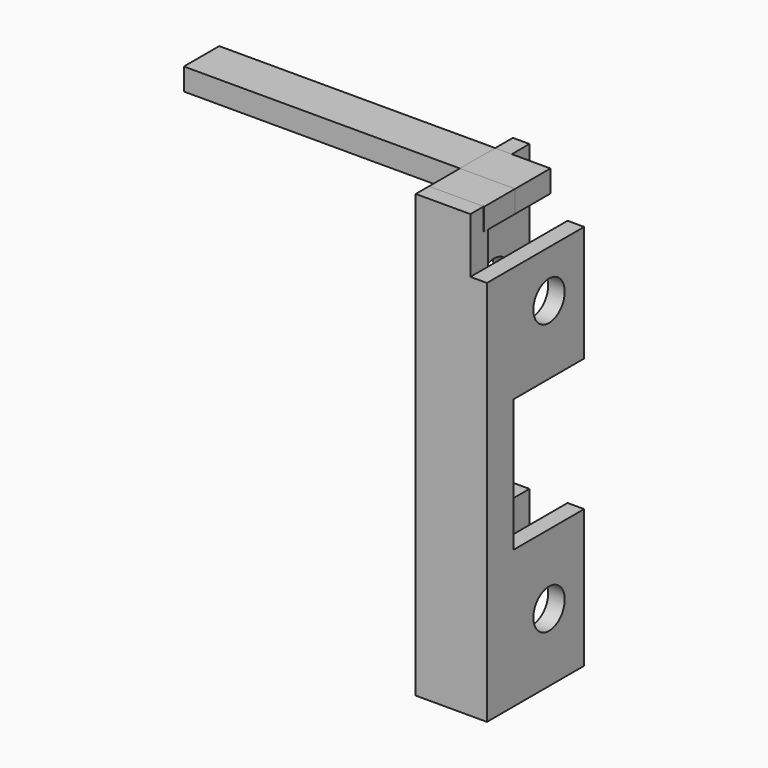
from build123d import *

# Parameters (mm, degrees)
F1_DEPTH  = 70
F2_R      = 3.55
F3_DEPTH  = 12.901
F5_DEPTH  = 10
F6_W      = 8
F6_H      = 4
F7_DEPTH  = 50
F8_W      = 9.9
F8_H      = 24
F8_W_2    = 3
F9_DEPTH  = 16
F10_DEPTH = 10
F11_DEPTH = 7


# Not quite as in the source:
# - a feature names something its author has since deleted; it is built from what else it names


with BuildPart() as f1:
    # F0 (on Top) → F1 (new body)
    with BuildSketch(Plane.XY):
        Polygon((0, 22), (0, 0), (12.9, 0), (12.9, 22), (9.9, 22), (9.9, 4), (3, 4), (3, 22), align=None)
    extrude(amount=F1_DEPTH)

    # F2 (on face) → F3 (cut, through all)
    with BuildSketch(Plane.YZ.offset(12.9)):
        with Locations((14.05, 61.45)):
            Circle(F2_R)
        with Locations((14.05, 12.35)):
            Circle(F2_R)
    extrude(amount=-F3_DEPTH, mode=Mode.SUBTRACT)

    # F4 (on face) → F5 (join)
    with BuildSketch(Plane.XY.offset(70)):
        Polygon((9.9, 0), (9.9, 4), (3, 4), (3, 22), (0, 22), (0, 0), align=None)
    extrude(amount=F5_DEPTH)

    # F8 (on face) → F9 (cut)
    with BuildSketch(Plane(origin=(0, 22, 0), x_dir=(-1, 0, 0), z_dir=(0, 1, 0))):
        with Locations((-4.95, 37)):
            Rectangle(F8_W, F8_H)
        with Locations((-11.4, 37)):
            Rectangle(F8_W_2, F8_H)
    extrude(amount=-F9_DEPTH, mode=Mode.SUBTRACT)


with BuildPart() as f7:
    # F6 (on face) → F7 (new body)
    with BuildSketch(Plane(origin=(0, 0, 0), x_dir=(0, -1, 0), z_dir=(-1, 0, 0))):
        with Locations((-14, 78)):
            Rectangle(F6_W, F6_H)
    extrude(amount=F7_DEPTH)


with BuildPart() as f10:
    # F6 (on face) → F10 (new body)
    with BuildSketch(Plane(origin=(0, 0, 0), x_dir=(0, -1, 0), z_dir=(-1, 0, 0))):
        with Locations((-14, 78)):
            Rectangle(F6_W, F6_H)
    extrude(amount=-F10_DEPTH)


with BuildPart() as f11:
    # F11 (new): a face of the model
    f11_faces = [f10.part.faces().sort_by_distance(p)[0] for p in [
        (5, 10, 78),
    ]]
    extrude(f11_faces, amount=F11_DEPTH)


solid = Compound([f1.part, f7.part, f10.part, f11.part])
